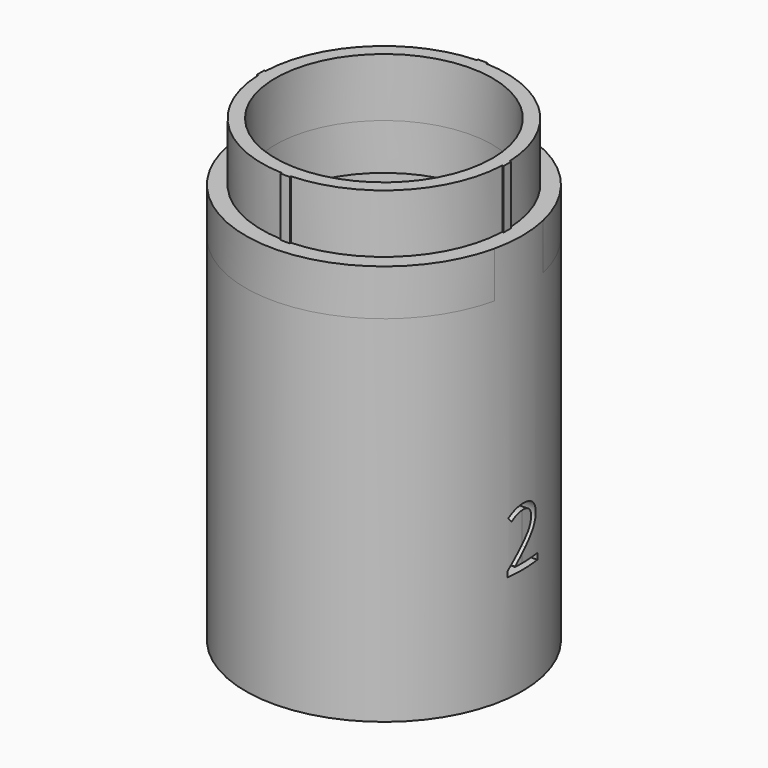
from build123d import *

# Parameters (mm, degrees)
F0_R         = 11.775
F1_DEPTH     = 6.35
F2_R         = 15
F2_R_2       = 13.4
F3_DEPTH     = 43.5
F4_R         = 15
F4_R_2       = 11.775
F5_DEPTH     = 5
F6_TEXT_SIZE = 8.7370552743
F7_DEPTH     = 25


# Not quite as in the source:
# - Text() gives the source's letters only with a copy of the font that has no kerning and outlines rounded to 1/6400 em; it was checked with that copy


with BuildPart() as f1:
    # F0 (on Top) → F1 (new body)
    with BuildSketch(Plane.XY):
        with BuildLine():
            ThreePointArc((13.2405626769, -0.5), (13.2476404591, -0.2500445276), (13.25, 0))
            ThreePointArc((13.25, 0), (13.2476404591, 0.2500445276), (13.2405626769, 0.5))
            ThreePointArc((13.2405626769, 0.5), (9.3691648507, 9.3691648507), (0.5, 13.2405626769))
            ThreePointArc((0.5, 13.2405626769), (0, 13.25), (-0.5, 13.2405626769))
            ThreePointArc((-0.5, 13.2405626769), (-9.3691648507, 9.3691648507), (-13.2405626769, 0.5))
            ThreePointArc((-13.2405626769, 0.5), (-13.25, 0), (-13.2405626769, -0.5))
            ThreePointArc((-13.2405626769, -0.5), (-9.3691648507, -9.3691648507), (-0.5, -13.2405626769))
            ThreePointArc((-0.5, -13.2405626769), (0, -13.25), (0.5, -13.2405626769))
            ThreePointArc((0.5, -13.2405626769), (9.3691648507, -9.3691648507), (13.2405626769, -0.5))
        make_face()
        Circle(F0_R, mode=Mode.SUBTRACT)
        with BuildLine():
            ThreePointArc((13.2405626769, 0.5), (13.2476404591, 0.2500445276), (13.25, 0))
            ThreePointArc((13.25, 0), (13.2476404591, -0.2500445276), (13.2405626769, -0.5))
            Line((13.2405626769, -0.5), (13.3906683926, -0.5))
            ThreePointArc((13.3906683926, -0.5), (13.4, 0), (13.3906683926, 0.5))
            Line((13.3906683926, 0.5), (13.2405626769, 0.5))
        make_face()
        with BuildLine():
            ThreePointArc((-0.5, 13.2405626769), (0, 13.25), (0.5, 13.2405626769))
            Line((0.5, 13.2405626769), (0.5, 13.3906683926))
            ThreePointArc((0.5, 13.3906683926), (0, 13.4), (-0.5, 13.3906683926))
            Line((-0.5, 13.3906683926), (-0.5, 13.2405626769))
        make_face()
        with BuildLine():
            Line((0.5, -13.3906683926), (0.5, -13.2405626769))
            ThreePointArc((0.5, -13.2405626769), (0, -13.25), (-0.5, -13.2405626769))
            Line((-0.5, -13.2405626769), (-0.5, -13.3906683926))
            ThreePointArc((-0.5, -13.3906683926), (0, -13.4), (0.5, -13.3906683926))
        make_face()
        with BuildLine():
            ThreePointArc((-13.2405626769, -0.5), (-13.25, 0), (-13.2405626769, 0.5))
            Line((-13.2405626769, 0.5), (-13.3906683926, 0.5))
            ThreePointArc((-13.3906683926, 0.5), (-13.4, 0), (-13.3906683926, -0.5))
            Line((-13.3906683926, -0.5), (-13.2405626769, -0.5))
        make_face()
    extrude(amount=F1_DEPTH)

    # F2 (on Top) → F3 (join)
    with BuildSketch(Plane.XY):
        Circle(F2_R)
        Circle(F2_R_2, mode=Mode.SUBTRACT)
    extrude(amount=-F3_DEPTH)

    # F6 (on Right) → F7 (cut)
    with BuildSketch(Plane.YZ):
        with Locations((-2.263443382, -31.9193787873)):
            Text('2', F6_TEXT_SIZE, font='Open Sans', text_align=(TextAlign.LEFT, TextAlign.BOTTOM))
    extrude(amount=F7_DEPTH, mode=Mode.SUBTRACT)


with BuildPart() as f5:
    # F4 (on Top) → F5 (new body)
    with BuildSketch(Plane.XY):
        Circle(F4_R)
        Circle(F4_R_2, mode=Mode.SUBTRACT)
    extrude(amount=-F5_DEPTH)


solid = Compound([f1.part, f5.part])
